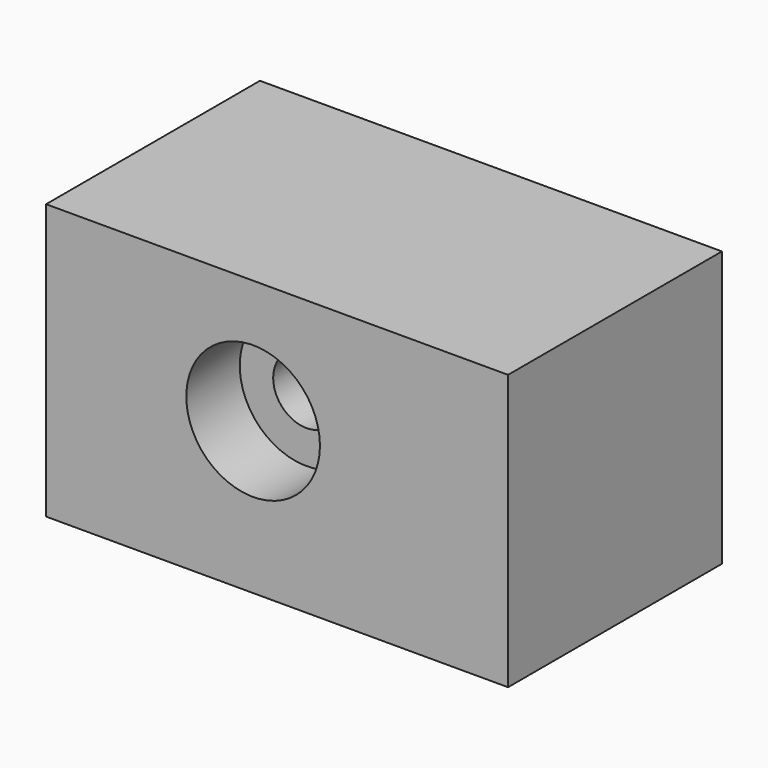
from build123d import *

# Parameters (mm, degrees)
F0_W           = 43.89539361
F0_H           = 26.1317063123
F1_DEPTH       = 25.4
F3_D           = 6.35
F3_DEPTH       = 12.7
F3_CBORE_D     = 12.7
F3_CBORE_DEPTH = 6.35
F3_TIP         = 1.9077324654


with BuildPart() as f1:
    # F0 (on Front) → F1 (new body)
    with BuildSketch(Plane.XZ):
        with Locations((-21.947696805, 13.0658531561)):
            Rectangle(F0_W, F0_H)
    extrude(amount=F1_DEPTH)

    # F3
    with Locations(Plane.XZ.offset(25.4)):
        with Locations((-24.2232121527, 14.3871195614)):
            CounterBoreHole(F3_D / 2, F3_CBORE_D / 2, F3_CBORE_DEPTH, depth=F3_DEPTH)
            with Locations((0, 0, -(F3_DEPTH + F3_TIP / 2))):  # 118° drill point
                Cone(0, F3_D / 2, F3_TIP, mode=Mode.SUBTRACT)


solid = f1.part
